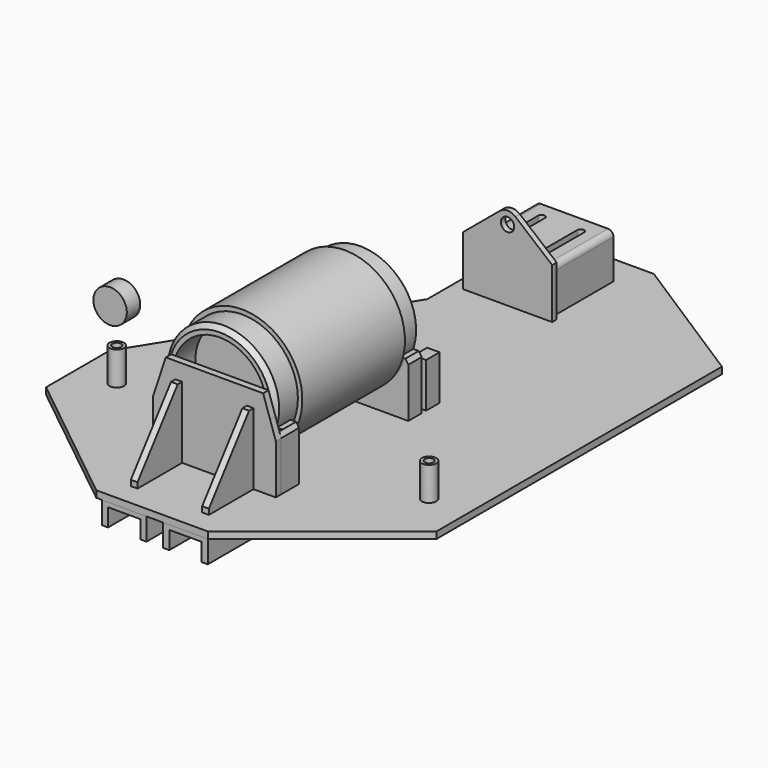
from build123d import *

# Parameters (mm, degrees)
F0_R           = 50
F1_DEPTH       = 25
F2_R           = 54
F2_R_2         = 50
F3_DEPTH       = 115
F4_R           = 50
F5_DEPTH       = 17.5
F6_R           = 42
F7_DEPTH       = 25
F9_R           = 15
F9_R_2         = 13.5
F10_DEPTH      = 15
F12_DEPTH      = 15
F13_DEPTH      = 15
F17_START      = 5
F17_DEPTH      = 20
F20_DEPTH      = 6
F24_DEPTH      = 20
F25_W          = 110
F25_H          = 20
F26_DEPTH      = 6
F29_SIZE       = 4
F32_DEPTH      = 70
F33_R          = 5
F35_DEPTH      = 25
F35_DEPTH_BACK = 25
F36_SIZE       = 5
F37_R          = 6.5
F37_R_2        = 4
F38_DEPTH      = 30
F39_ANGLE      = 180
F41_R          = 6
F42_DEPTH      = 5
F44_DEPTH      = 500
F47_DEPTH      = 6
F49_DEPTH      = 6
F52_DEPTH      = 5


with BuildPart() as f1:
    # F0 (on Front) → F1 (new body)
    with BuildSketch(Plane.XZ):
        Circle(F0_R)
    extrude(amount=-F1_DEPTH)

    # F2 (on face) → F3 (join)
    with BuildSketch(Plane(origin=(0, 25, 0), x_dir=(-1, 0, 0), z_dir=(0, 1, 0))):
        Circle(F2_R)
        Circle(F2_R_2, mode=Mode.SUBTRACT)
        Circle(F2_R_2)
    extrude(amount=F3_DEPTH)

    # F4 (on face) → F5 (join)
    with BuildSketch(Plane(origin=(0, 140, 0), x_dir=(-1, 0, 0), z_dir=(0, 1, 0))):
        Circle(F4_R)
    extrude(amount=F5_DEPTH)

    # F6 (on face) → F7 (cut)
    with BuildSketch(Plane.XZ):
        Circle(F6_R)
    extrude(amount=-F7_DEPTH, mode=Mode.SUBTRACT)

    # F29
    f29_edges = [f1.edges().sort_by_distance(p)[0] for p in [
        (-50, 0, 0),
    ]]
    chamfer(f29_edges, length=F29_SIZE)


with BuildPart() as f10:
    # F9 (on offset) → F10 (new body)
    with BuildSketch(Plane.XZ.offset(-52)):
        with Locations((-140, 0)):
            Circle(F9_R)
        with Locations((-140, 0)):
            Circle(F9_R_2, mode=Mode.SUBTRACT)
        with Locations((-140, 0)):
            Circle(F9_R_2)
    extrude(amount=-F10_DEPTH)


with BuildPart() as f12:
    # F11 (on face) → F12 (new body)
    with BuildSketch(Plane(origin=(0, 157.5, 0), x_dir=(-1, 0, 0), z_dir=(0, 1, 0))):
        with BuildLine():
            ThreePointArc((47.4755537034, -15.6866758924), (0, -50), (-47.4755537034, -15.6866758924))
            Line((-47.4755537034, -15.6866758924), (-51.6713479546, -15.6866758924))
            ThreePointArc((-51.6713479546, -15.6866758924), (0, -54), (51.6713479546, -15.6866758924))
            Line((51.6713479546, -15.6866758924), (47.4755537034, -15.6866758924))
        make_face()
    extrude(amount=-F12_DEPTH)


with BuildPart() as f13:
    # F11 (on face) → F13 (new body)
    with BuildSketch(Plane(origin=(0, 157.5, 0), x_dir=(-1, 0, 0), z_dir=(0, 1, 0))):
        with BuildLine():
            ThreePointArc((51.6713479546, -15.6866758924), (0, -54), (-51.6713479546, -15.6866758924))
            Line((-51.6713479546, -15.6866758924), (-52.3915120419, -15.6866758924))
            Line((-52.3915120419, -15.6866758924), (-55, -19.6446609407))
            Line((-55, -19.6446609407), (-55, -64))
            Line((-55, -64), (0, -64))
            Line((0, -64), (55, -64))
            Line((55, -64), (55, -19.6446609407))
            Line((55, -19.6446609407), (52.3915120419, -15.6866758924))
            Line((52.3915120419, -15.6866758924), (51.6713479546, -15.6866758924))
        make_face()
    extrude(amount=-F13_DEPTH)


with BuildPart() as f14_1:
    # F14: copy of F12
    add(f12.part.moved(Location((0, -137.5, 0))))


with BuildPart() as f17:
    # F16 (on face) → F17 (new body)
    with BuildSketch(Plane.XZ.offset(-25).offset(F17_START)):
        with BuildLine():
            Line((-55, -19.6446609407), (-55, -64))
            Line((-55, -64), (0, -64))
            Line((0, -64), (55, -64))
            Line((55, -64), (55, -19.6446609407))
            Line((55, -19.6446609407), (52.3915120419, -15.6866758924))
            Line((52.3915120419, -15.6866758924), (51.6713479546, -15.6866758924))
            ThreePointArc((51.6713479546, -15.6866758924), (0, -54), (-51.6713479546, -15.6866758924))
            Line((-51.6713479546, -15.6866758924), (-52.3915120419, -15.6866758924))
            Line((-52.3915120419, -15.6866758924), (-55, -19.6446609407))
        make_face()
    extrude(amount=F17_DEPTH)


with BuildPart() as f20:
    # F19 (on offset) → F20 (new body)
    with BuildSketch(Plane.YZ.offset(35)):
        Polygon((-6, -19.6446609407), (-6, 0), (-11, 0), (-56, -59), (-56, -64), (-6, -64), align=None)
    extrude(amount=-F20_DEPTH)


with BuildPart() as f21_1:
    # F21: copy of F20
    add(f20.part.moved(Location((-64, 0, 0))))


with BuildPart() as f24:
    # F23 (on offset) → F24 (new body)
    with BuildSketch(Plane(origin=(0, 182.5, 0), x_dir=(-1, 0, 0), z_dir=(0, 1, 0))):
        with BuildLine():
            ThreePointArc((43.8634243989, -24), (0, -50), (-43.8634243989, -24))
            Line((-43.8634243989, -24), (-55, -24))
            Line((-55, -24), (-55, -64))
            Line((-55, -64), (0, -64))
            Line((0, -64), (55, -64))
            Line((55, -64), (55, -24))
            Line((55, -24), (43.8634243989, -24))
        make_face()
    extrude(amount=-F24_DEPTH)

    # F23 (on offset) → F52 (cut)
    with BuildSketch(Plane(origin=(0, 182.5, 0), x_dir=(-1, 0, 0), z_dir=(0, 1, 0))):
        with BuildLine():
            ThreePointArc((43.8634243989, -24), (0, -50), (-43.8634243989, -24))
            Line((-43.8634243989, -24), (-55, -24))
            Line((-55, -24), (-55, -64))
            Line((-55, -64), (0, -64))
            Line((0, -64), (55, -64))
            Line((55, -64), (55, -24))
            Line((55, -24), (43.8634243989, -24))
        make_face()
    extrude(amount=-F52_DEPTH, mode=Mode.SUBTRACT)


with BuildPart() as f26:
    # F25 (on face) → F26 (new body)
    with BuildSketch(Plane(origin=(0, 0, -64), x_dir=(1, 0, 0), z_dir=(0, 0, -1))):
        Polygon((-50, 76), (-175, -24), (-175, -95), (-50, -295), (-50, -424), (50, -424), (50, -295), (175, -95), (175, -24), (50, 76), align=None)
        with Locations((0, -10)):
            Rectangle(F25_W, F25_H, mode=Mode.SUBTRACT)
        with Locations((0, -10)):
            Rectangle(F25_W, F25_H)
    extrude(amount=F26_DEPTH)

    # F36
    f36_edges = [f26.edges().sort_by_distance(p)[0] for p in [
        (-50, 424, -67),
    ]]
    chamfer(f36_edges, length=F36_SIZE)

    # F48 (on face) → F49 (join, through all)
    with BuildSketch(Plane(origin=(0, 0, -70), x_dir=(1, 0, 0), z_dir=(0, 0, -1))):
        Polygon((175, -344), (175, -95), (50, -295), (50, -424), align=None)
    extrude(amount=-F49_DEPTH)


with BuildPart() as f32:
    # F31 (on offset) → F32 (new body)
    with BuildSketch(Plane(origin=(0, 327.5, 0), x_dir=(-1, 0, 0), z_dir=(0, 1, 0))):
        Polygon((-35, -24), (-35, -64), (-30, -64), (-30, -29), (30, -29), (30, -64), (35, -64), (35, -24), align=None)
    extrude(amount=F32_DEPTH)

    # F33
    f33_edges = [f32.edges().sort_by_distance(p)[0] for p in [
        (35, 362.5, -24),
        (-35, 362.5, -24),
        (-30, 362.5, -29),
        (30, 362.5, -29),
    ]]
    fillet(f33_edges, radius=F33_R)

    # F34 (on face) → F35 (cut, two sides)
    with BuildSketch(Plane.XY.offset(-24)) as f35_sk:
        with BuildLine():
            Line((-20.5, 382.5), (-20.5, 342.5))
            ThreePointArc((-20.5, 342.5), (-17.5, 339.5), (-14.5, 342.5))
            Line((-14.5, 342.5), (-14.5, 382.5))
            ThreePointArc((-14.5, 382.5), (-17.5, 385.5), (-20.5, 382.5))
        make_face()
        with BuildLine():
            Line((14.5, 382.5), (14.5, 342.5))
            ThreePointArc((14.5, 342.5), (17.5, 339.5), (20.5, 342.5))
            Line((20.5, 342.5), (20.5, 382.5))
            ThreePointArc((20.5, 382.5), (17.5, 385.5), (14.5, 382.5))
        make_face()
    extrude(amount=-F35_DEPTH, mode=Mode.SUBTRACT)
    extrude(f35_sk.sketch, amount=F35_DEPTH_BACK, mode=Mode.SUBTRACT)


with BuildPart() as f38:
    # F37 (on face) → F38 (new body)
    with BuildSketch(Plane.XY.offset(-64)):
        with Locations((-140, 59.5)):
            Circle(F37_R)
        with Locations((-140, 59.5)):
            Circle(F37_R_2, mode=Mode.SUBTRACT)
    extrude(amount=F38_DEPTH)


with BuildPart() as f39_1:
    # F39: copy of F38
    add(f38.part.rotate(Axis((0, 59.5, -50), (0, 0, -1)), F39_ANGLE))


with BuildPart() as f42:
    # F41 (on offset) → F42 (new body)
    with BuildSketch(Plane(origin=(0, 327.5, 0), x_dir=(-1, 0, 0), z_dir=(0, 1, 0))):
        with BuildLine():
            Line((-40, -64), (40, -64))
            Line((40, -64), (40, -19))
            Line((40, -19), (7.0398272445, 8.4522678831))
            ThreePointArc((7.0398272445, 8.4522678831), (0, 11), (-7.0398272445, 8.4522678831))
            Line((-7.0398272445, 8.4522678831), (-40, -19))
            Line((-40, -19), (-40, -64))
        make_face()
        Circle(F41_R, mode=Mode.SUBTRACT)
    extrude(amount=-F42_DEPTH)


with BuildPart() as f44:
    # F43 (on face) → F44 (new body, through all)
    with BuildSketch(Plane.XZ.offset(76)):
        Polygon((50, -90), (50, -70), (10, -70), (10, -90), (15.5, -90), (15.5, -74), (44.5, -74), (44.5, -90), align=None)
    extrude(amount=-F44_DEPTH)


with BuildPart() as f45_1:
    # F45: copy of F44
    add(f44.part.moved(Location((-60, 0, 0))))


with BuildPart() as f47:
    # F46 (on face) → F47 (new body)
    with BuildSketch(Plane.XZ):
        with BuildLine():
            Line((-55, -19.6446609407), (-55, -64))
            Line((-55, -64), (55, -64))
            Line((55, -64), (55, -19.6446609407))
            Line((55, -19.6446609407), (49.832295564, -4.0917378732))
            ThreePointArc((49.832295564, -4.0917378732), (0, -50), (-49.832295564, -4.0917378732))
            Line((-49.832295564, -4.0917378732), (-55, -19.6446609407))
        make_face()
        with BuildLine():
            Line((-43.6533919821, 14.5045292395), (-49.832295564, -4.0917378732))
            ThreePointArc((-49.832295564, -4.0917378732), (0, -50), (49.832295564, -4.0917378732))
            Line((49.832295564, -4.0917378732), (43.6533919821, 14.5045292395))
            Line((43.6533919821, 14.5045292395), (-43.6533919821, 14.5045292395))
        make_face()
    extrude(amount=F47_DEPTH)


with BuildPart() as f45_1_1:
    # F50: moved
    add(f45_1.part.moved(Location((5, 0, 0))))


solid = Compound([f1.part, f10.part, f12.part, f13.part, f14_1.part, f17.part, f20.part, f21_1.part, f24.part, f26.part, f32.part, f38.part, f39_1.part, f42.part, f44.part, f47.part, f45_1_1.part])
